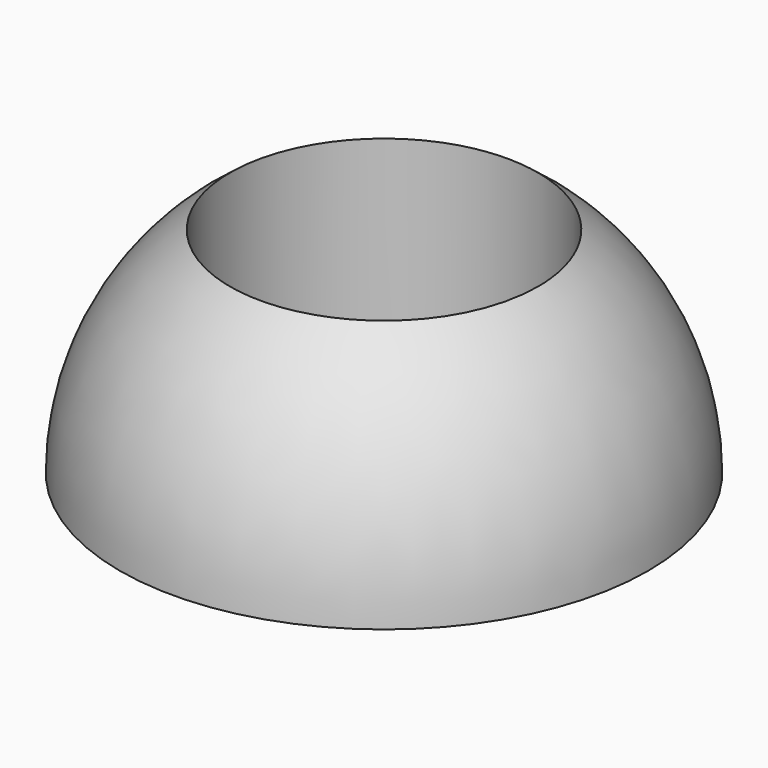
from build123d import *

# Parameters (mm, degrees)
F0_R     = 38.1
F1_DEPTH = 38.1
F2_R     = 38.09999
F3_R     = 22.225
F4_DEPTH = 151.384


# Not quite as in the source:
# - a fillet or chamfer is up to 0.001 mm smaller than in the source, because OpenCascade refuses the exact size


with BuildPart() as f1:
    # F0 (on Top) → F1 (new body)
    with BuildSketch(Plane.XY):
        Circle(F0_R)
    extrude(amount=F1_DEPTH)

    # F2 (radius 38.1 in the source; OpenCascade refuses exactly that, so slightly less here)
    f2_edges = [f1.edges().sort_by_distance(p)[0] for p in [
        (-38.1, 0, 38.1),
    ]]
    fillet(f2_edges, radius=F2_R)

    # F3 (on Top) → F4 (cut)
    with BuildSketch(Plane.XY):
        Circle(F3_R)
    extrude(amount=F4_DEPTH, mode=Mode.SUBTRACT)


solid = f1.part
